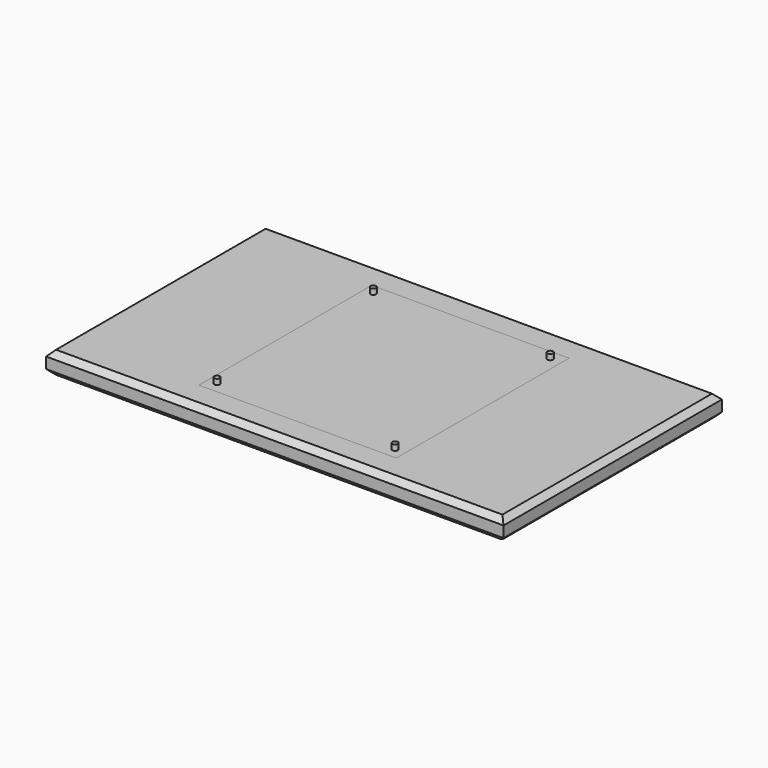
from build123d import *

# Parameters (mm, degrees)
F0_W        = 248
F0_H        = 148
F1_DEPTH    = 12
F2_SIZE     = 3
F3_T1_DEPTH = 163.4300979278
F3_T3_DEPTH = 260.4300979278
F3_T5_DEPTH = 154.7714251613
F4_W        = 56.3140325248
F4_H        = 92.5788208842
F5_DEPTH    = 1
F6_W        = 106.9637537003
F6_H        = 117.1658635139
F7_DEPTH    = 4
F8_W        = 106.9637537003
F8_H        = 117.1658635139
F9_DEPTH    = 4
F10_R       = 1.5
F11_DEPTH   = 3
F17_SIZE    = 3


# Not quite as in the source:
# - a fillet or chamfer that OpenCascade refuses, or shapes differently, is made with other operations: its cross-section is extruded or revolved along the edge and cut away or added


with BuildPart() as f1:
    # F0 (on Top) → F1 (new body)
    with BuildSketch(Plane.XY):
        Rectangle(F0_W, F0_H)
    extrude(amount=F1_DEPTH)

    # F2
    f2_edges = [f1.edges().sort_by_distance(p)[0] for p in [
        (0, 74, 12),
        (-124, 0, 12),
        (0, -74, 12),
        (124, 0, 0),
    ]]
    chamfer(f2_edges, length=F2_SIZE)

    # F3: chamfer of 3 on 4 edges, made by hand

    # F3_s2 → F3_t1 (cut)
    with BuildSketch(Plane.XZ.offset(-81.7150489639)):
        Polygon((-124, 3), (-121, 0), (-124, 0), align=None)
    extrude(amount=F3_T1_DEPTH, mode=Mode.SUBTRACT)

    # F3_s4 → F3_t3 (cut)
    with BuildSketch(Plane.YZ.offset(-131.7150489639)):
        Polygon((74, 3), (71, 0), (74, 0), align=None)
        Polygon((-71, 0), (-74, 3), (-74, 0), align=None)
    extrude(amount=F3_T3_DEPTH, mode=Mode.SUBTRACT)

    # F3_s6 → F3_t5 (cut)
    with BuildSketch(Plane.XZ.offset(-77.3857125806)):
        Polygon((119.7573593129, 0), (121.8786796564, 0.8786796564), (121, 0), align=None)
    extrude(amount=F3_T5_DEPTH, mode=Mode.SUBTRACT)

    # F6 (on face) → F7 (cut)
    with BuildSketch(Plane.XY.offset(12)):
        Rectangle(F6_W, F6_H)
    extrude(amount=-F7_DEPTH, mode=Mode.SUBTRACT)

    # F17
    f17_edges = [f1.edges().sort_by_distance(p)[0] for p in [
        (124, 0, 12),
    ]]
    chamfer(f17_edges, length=F17_SIZE)


with BuildPart() as f5:
    # F4 (on Top) → F5 (new body)
    with BuildSketch(Plane.XY):
        Rectangle(F4_W, F4_H)
    extrude(amount=-F5_DEPTH)


with BuildPart() as f9:
    # F8 (on face) → F9 (new body)
    with BuildSketch(Plane.XY.offset(8)):
        Rectangle(F8_W, F8_H)
    extrude(amount=F9_DEPTH)


with BuildPart() as f11:
    # F10 (on face) → F11 (new body)
    with BuildSketch(Plane.XY.offset(12)):
        with Locations((-48.4135895967, 53.2953217626)):
            Circle(F10_R)
    extrude(amount=F11_DEPTH)


with BuildPart() as f12_1:
    # F12: copy of F11
    add(f11.part)


with BuildPart() as f14_1:
    # F14: copy of F11
    add(f11.part.moved(Location((95.9, 0, 0))))


with BuildPart() as f15_1:
    # F15: copy of F11
    add(f11.part.moved(Location((0, -105.9, 0))))


with BuildPart() as f16_1:
    # F16: copy of F15_1
    add(f15_1.part.moved(Location((96.5, 0, 0))))


solid = Compound([f1.part, f5.part, f9.part, f11.part, f14_1.part, f15_1.part, f16_1.part])
